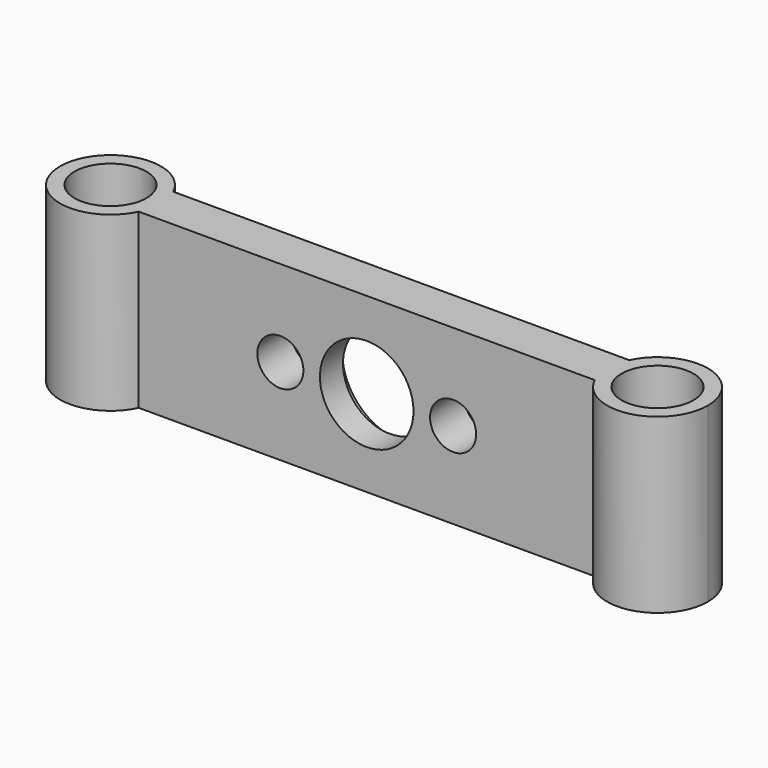
from build123d import *

# Parameters (mm, degrees)
F1_DEPTH       = 12
F2_D           = 5
F2_DEPTH       = 15
F2_TIP         = 1.5021515476
F3_D           = 5
F3_DEPTH       = 15
F3_TIP         = 1.5021515476
F5_D           = 6.5
F5_DEPTH       = 10
F5_CBORE_D     = 8.2
F5_CBORE_DEPTH = 1
F5_TIP         = 1.9527970118
F6_D           = 3.2
F6_DEPTH       = 15
F6_TIP         = 0.9613769904
F7_D           = 3.2
F7_DEPTH       = 15
F7_TIP         = 0.9613769904


# Not quite as in the source:
# - a feature names something its author has since deleted; it is built from what else it names


with BuildPart() as f1:
    # F0 (on Top) → F1 (new body)
    with BuildSketch(Plane.XY):
        with BuildLine():
            Line((-19, -1.8754155822), (-19, 1.1245844178))
            Line((-19, 1.1245844178), (-15.8377223398, 1.1245844178))
            ThreePointArc((-15.8377223398, 1.1245844178), (-22.5, -0.3754155822), (-15.8377223398, -1.8754155822))
            Line((-15.8377223398, -1.8754155822), (-19, -1.8754155822))
        make_face()
        with BuildLine():
            Line((-15.8377223398, 1.1245844178), (-19, 1.1245844178))
            Line((-19, 1.1245844178), (-19, -1.8754155822))
            Line((-19, -1.8754155822), (-15.8377223398, -1.8754155822))
            ThreePointArc((-15.8377223398, -1.8754155822), (-15.5854742781, -1.144189993), (-15.5, -0.3754155822))
            ThreePointArc((-15.5, -0.3754155822), (-15.5854742781, 0.3933588286), (-15.8377223398, 1.1245844178))
        make_face()
        with BuildLine():
            Line((15.8377223398, 1.1245844178), (-15.8377223398, 1.1245844178))
            ThreePointArc((-15.8377223398, 1.1245844178), (-15.5854742781, 0.3933588286), (-15.5, -0.3754155822))
            ThreePointArc((-15.5, -0.3754155822), (-15.5854742781, -1.144189993), (-15.8377223398, -1.8754155822))
            Line((-15.8377223398, -1.8754155822), (15.8377223398, -1.8754155822))
            ThreePointArc((15.8377223398, -1.8754155822), (15.5, -0.3754155822), (15.8377223398, 1.1245844178))
        make_face()
        with BuildLine():
            ThreePointArc((22.5, -0.3754155822), (19.7687744108, 3.0391101397), (15.8377223398, 1.1245844178))
            Line((15.8377223398, 1.1245844178), (19, 1.1245844178))
            Line((19, 1.1245844178), (19, -1.8754155822))
            Line((19, -1.8754155822), (15.8377223398, -1.8754155822))
            ThreePointArc((15.8377223398, -1.8754155822), (19.7687744108, -3.7899413041), (22.5, -0.3754155822))
        make_face()
        with BuildLine():
            Line((19, 1.1245844178), (15.8377223398, 1.1245844178))
            ThreePointArc((15.8377223398, 1.1245844178), (15.5, -0.3754155822), (15.8377223398, -1.8754155822))
            Line((15.8377223398, -1.8754155822), (19, -1.8754155822))
            Line((19, -1.8754155822), (19, 1.1245844178))
        make_face()
    extrude(amount=F1_DEPTH)

    # F2
    with Locations(Plane(origin=(0, 0, 0), x_dir=(1, 0, 0), z_dir=(0, 0, -1))):
        with Locations((19, 0.3754155822)):
            Hole(F2_D / 2, depth=F2_DEPTH)
            with Locations((0, 0, -(F2_DEPTH + F2_TIP / 2))):  # 118° drill point
                Cone(0, F2_D / 2, F2_TIP, mode=Mode.SUBTRACT)

    # F3
    with Locations(Plane(origin=(0, 0, 0), x_dir=(1, 0, 0), z_dir=(0, 0, -1))):
        with Locations((-19, 0.3754155822)):
            Hole(F3_D / 2, depth=F3_DEPTH)
            with Locations((0, 0, -(F3_DEPTH + F3_TIP / 2))):  # 118° drill point
                Cone(0, F3_D / 2, F3_TIP, mode=Mode.SUBTRACT)

    # F5
    with Locations(Plane(origin=(0, 1.1245844178, 0), x_dir=(-1, 0, 0), z_dir=(0, 1, 0))):
        with Locations((0, 6)):
            CounterBoreHole(F5_D / 2, F5_CBORE_D / 2, F5_CBORE_DEPTH, depth=F5_DEPTH)
            with Locations((0, 0, -(F5_DEPTH + F5_TIP / 2))):  # 118° drill point
                Cone(0, F5_D / 2, F5_TIP, mode=Mode.SUBTRACT)

    # F6
    with Locations(Plane(origin=(0, 1.1245844178, 0), x_dir=(-1, 0, 0), z_dir=(0, 1, 0))):
        with Locations((-6, 6)):
            Hole(F6_D / 2, depth=F6_DEPTH)
            with Locations((0, 0, -(F6_DEPTH + F6_TIP / 2))):  # 118° drill point
                Cone(0, F6_D / 2, F6_TIP, mode=Mode.SUBTRACT)

    # F7
    with Locations(Plane(origin=(0, 1.1245844178, 0), x_dir=(-1, 0, 0), z_dir=(0, 1, 0))):
        with Locations((6, 6)):
            Hole(F7_D / 2, depth=F7_DEPTH)
            with Locations((0, 0, -(F7_DEPTH + F7_TIP / 2))):  # 118° drill point
                Cone(0, F7_D / 2, F7_TIP, mode=Mode.SUBTRACT)


solid = f1.part
